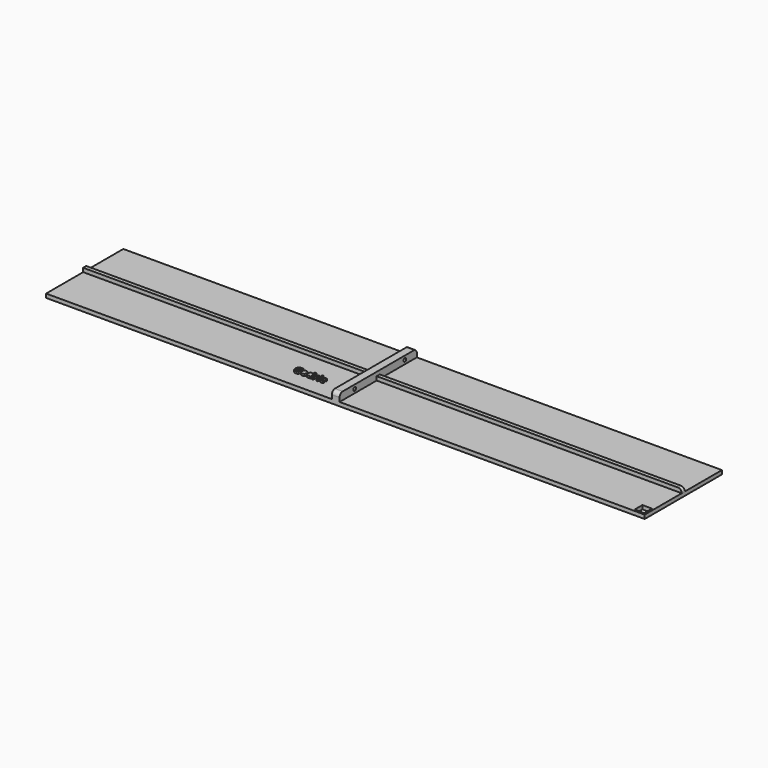
from build123d import *

# Parameters (mm, degrees)
F1_DEPTH     = 2
F0_W         = 0.7426452889
F0_H         = 2.7227729689
F0_W_2       = 5
F0_H_2       = 5
F2_DEPTH     = 4
F3_DEPTH     = 6
F4_R         = 0.885
F5_DEPTH     = 30.275
F6_R         = 2
F0_TEXT_SIZE = 4.9873345738
F7_DEPTH     = 3


# Not quite as in the source:
# - Text() gives the source's letters only with a copy of the font that has no kerning and outlines rounded to 1/6400 em; it was checked with that copy


with BuildPart() as f1:
    # F0 (on Top) → F1 (new body)
    with BuildSketch(Plane.XY):
        Polygon((-87.8959557414, 31.1546225101), (-235.8959557414, 31.1546225101), (-235.8959557414, 7.1546225101), (-234.8959557414, 7.1546225101), (-87.8959557414, 7.1546225101), align=None)
    extrude(amount=F1_DEPTH)



with BuildPart() as f1b:
    # F0 (on Top) → F1, piece 2 (new body)
    with BuildSketch(Plane.XY):
        Polygon((74.1040442586, 31.1546225101), (-83.8959557414, 31.1546225101), (-83.8959557414, 7.1546225101), (64.1040442586, 7.1546225101), (74.1040442586, 7.1546225101), align=None)
    extrude(amount=F1_DEPTH)



with BuildPart() as f1c:
    # F0 (on Top) → F1, piece 3 (new body)
    with BuildSketch(Plane.XY):
        Polygon((-234.8959557414, 5.1546225101), (-235.8959557414, 5.1546225101), (-235.8959557414, -18.8453774899), (-87.8959557414, -18.8453774899), (-87.8959557414, 5.1546225101), align=None)
        with BuildLine():
            add(Edge.make_bspline(
                [(-109.0030381923, -8.150502003), (-108.8425083607, -8.4696134887), (-108.8425083607, -8.8982125536)],
                knots=[0, 0, 0, 1, 1, 1], degree=2))
            add(Edge.make_bspline(
                [(-108.8425083607, -8.8982125536), (-108.8425083607, -9.5629307398), (-109.1931803229, -9.9381497394)],
                knots=[0, 0, 0, 1, 1, 1], degree=2))
            add(Edge.make_bspline(
                [(-109.1931803229, -9.9381497394), (-109.5438522851, -10.3133687389), (-110.16960692, -10.3133687389)],
                knots=[0, 0, 0, 1, 1, 1], degree=2))
            add(Edge.make_bspline(
                [(-110.16960692, -10.3133687389), (-110.5615802466, -10.3133687389), (-110.8612099566, -10.1415394774)],
                knots=[0, 0, 0, 1, 1, 1], degree=2))
            add(Edge.make_bspline(
                [(-110.8612099566, -10.1415394774), (-111.1608396665, -9.969710216), (-111.3213694981, -9.6482609173)],
                knots=[0, 0, 0, 1, 1, 1], degree=2))
            add(Edge.make_bspline(
                [(-111.3213694981, -9.6482609173), (-111.4818993297, -9.3268116185), (-111.4818993297, -8.8982125536)],
                knots=[0, 0, 0, 1, 1, 1], degree=2))
            add(Edge.make_bspline(
                [(-111.4818993297, -8.8982125536), (-111.4818993297, -8.2311565544), (-111.1339548161, -7.8610028165)],
                knots=[0, 0, 0, 1, 1, 1], degree=2))
            add(Edge.make_bspline(
                [(-111.1339548161, -7.8610028165), (-110.7860103024, -7.4908490785), (-110.1548007704, -7.4908490785)],
                knots=[0, 0, 0, 1, 1, 1], degree=2))
            add(Edge.make_bspline(
                [(-110.1548007704, -7.4908490785), (-109.7628274438, -7.4908490785), (-109.4631977338, -7.661119798)],
                knots=[0, 0, 0, 1, 1, 1], degree=2))
            add(Edge.make_bspline(
                [(-109.4631977338, -7.661119798), (-109.1635680239, -7.8313905174), (-109.0030381923, -8.150502003)],
                knots=[0, 0, 0, 1, 1, 1], degree=2))
        make_face(mode=Mode.SUBTRACT)
        with BuildLine():
            Line((-113.5181345237, -8.8935369274), (-113.5181345237, -8.2646652085))
            Line((-113.5181345237, -8.2646652085), (-112.1053161514, -8.2646652085))
            Line((-112.1053161514, -8.2646652085), (-112.1053161514, -10.1107582719))
            add(Edge.make_bspline(
                [(-112.1053161514, -10.1107582719), (-112.4489746744, -10.2229732998), (-112.752111104, -10.2681710194)],
                knots=[0, 0, 0, 1, 1, 1], degree=2))
            add(Edge.make_bspline(
                [(-112.752111104, -10.2681710194), (-113.0552475335, -10.3133687389), (-113.3716315706, -10.3133687389)],
                knots=[0, 0, 0, 1, 1, 1], degree=2))
            add(Edge.make_bspline(
                [(-113.3716315706, -10.3133687389), (-114.1773978127, -10.3133687389), (-114.602490158, -9.8395719544)],
                knots=[0, 0, 0, 1, 1, 1], degree=2))
            add(Edge.make_bspline(
                [(-114.602490158, -9.8395719544), (-115.0275825033, -9.3657751699), (-115.0275825033, -8.478964741)],
                knots=[0, 0, 0, 1, 1, 1], degree=2))
            add(Edge.make_bspline(
                [(-115.0275825033, -8.478964741), (-115.0275825033, -7.6170909849), (-114.5343039431, -7.1351118546)],
                knots=[0, 0, 0, 1, 1, 1], degree=2))
            add(Edge.make_bspline(
                [(-114.5343039431, -7.1351118546), (-114.0410253829, -6.6531327243), (-113.1674625615, -6.6531327243)],
                knots=[0, 0, 0, 1, 1, 1], degree=2))
            add(Edge.make_bspline(
                [(-113.1674625615, -6.6531327243), (-112.6188557583, -6.6531327243), (-112.1099917776, -6.872107883)],
                knots=[0, 0, 0, 1, 1, 1], degree=2))
            Line((-112.1099917776, -6.872107883), (-112.3609170483, -7.476042929))
            add(Edge.make_bspline(
                [(-112.3609170483, -7.476042929), (-112.7505525619, -7.2812251722), (-113.1721381876, -7.2812251722)],
                knots=[0, 0, 0, 1, 1, 1], degree=2))
            add(Edge.make_bspline(
                [(-113.1721381876, -7.2812251722), (-113.6615203927, -7.2812251722), (-113.9560848409, -7.6100775457)],
                knots=[0, 0, 0, 1, 1, 1], degree=2))
            add(Edge.make_bspline(
                [(-113.9560848409, -7.6100775457), (-114.2506492892, -7.9389299192), (-114.2506492892, -8.4937708905)],
                knots=[0, 0, 0, 1, 1, 1], degree=2))
            add(Edge.make_bspline(
                [(-114.2506492892, -8.4937708905), (-114.2506492892, -9.0735485347), (-114.0133612614, -9.3790227774)],
                knots=[0, 0, 0, 1, 1, 1], degree=2))
            add(Edge.make_bspline(
                [(-114.0133612614, -9.3790227774), (-113.7760732337, -9.68449702), (-113.3233167669, -9.68449702)],
                knots=[0, 0, 0, 1, 1, 1], degree=2))
            add(Edge.make_bspline(
                [(-113.3233167669, -9.68449702), (-113.0864183746, -9.68449702), (-112.8432858142, -9.6361822163)],
                knots=[0, 0, 0, 1, 1, 1], degree=2))
            Line((-112.8432858142, -9.6361822163), (-112.8432858142, -8.8935369274))
            Line((-112.8432858142, -8.8935369274), (-113.5181345237, -8.8935369274))
        make_face(mode=Mode.SUBTRACT)
        with BuildLine():
            add(Edge.make_bspline(
                [(-104.0215481511, -7.6307282279), (-103.8060797121, -7.4908490785), (-103.5528166283, -7.4908490785)],
                knots=[0, 0, 0, 1, 1, 1], degree=2))
            add(Edge.make_bspline(
                [(-103.5528166283, -7.4908490785), (-103.401638049, -7.4908490785), (-103.3018913576, -7.5126686673)],
                knots=[0, 0, 0, 1, 1, 1], degree=2))
            Line((-103.3018913576, -7.5126686673), (-103.3579988715, -8.2085576946))
            add(Edge.make_bspline(
                [(-103.3579988715, -8.2085576946), (-103.4483943107, -8.1844002927), (-103.5769740301, -8.1844002927)],
                knots=[0, 0, 0, 1, 1, 1], degree=2))
            add(Edge.make_bspline(
                [(-103.5769740301, -8.1844002927), (-103.9323216185, -8.1844002927), (-104.1310357305, -8.3671393486)],
                knots=[0, 0, 0, 1, 1, 1], degree=2))
            add(Edge.make_bspline(
                [(-104.1310357305, -8.3671393486), (-104.3297498424, -8.5498784045), (-104.3297498424, -8.8787307779)],
                knots=[0, 0, 0, 1, 1, 1], degree=2))
            Line((-104.3297498424, -8.8787307779), (-104.3297498424, -10.2642746642))
            Line((-104.3297498424, -10.2642746642), (-105.0723951313, -10.2642746642))
            Line((-105.0723951313, -10.2642746642), (-105.0723951313, -7.5415016953))
            Line((-105.0723951313, -7.5415016953), (-104.5097614497, -7.5415016953))
            Line((-104.5097614497, -7.5415016953), (-104.3998842348, -7.9997130593))
            Line((-104.3998842348, -7.9997130593), (-104.3640377676, -7.9997130593))
            add(Edge.make_bspline(
                [(-104.3640377676, -7.9997130593), (-104.2370165902, -7.7706073773), (-104.0215481511, -7.6307282279)],
                knots=[0, 0, 0, 1, 1, 1], degree=2))
        make_face(mode=Mode.SUBTRACT)
        with Locations((-102.4365108819, -8.9028881798)):
            Rectangle(F0_W, F0_H, mode=Mode.SUBTRACT)
        with BuildLine():
            add(Edge.make_bspline(
                [(-99.7164653616, -10.2693399259), (-99.900373324, -10.3133687389), (-100.1801316227, -10.3133687389)],
                knots=[0, 0, 0, 1, 1, 1], degree=2))
            add(Edge.make_bspline(
                [(-100.1801316227, -10.3133687389), (-101.451122668, -10.3133687389), (-101.451122668, -8.9176943293)],
                knots=[0, 0, 0, 1, 1, 1], degree=2))
            add(Edge.make_bspline(
                [(-101.451122668, -8.9176943293), (-101.451122668, -8.2233638441), (-101.1055159675, -7.8571064613)],
                knots=[0, 0, 0, 1, 1, 1], degree=2))
            add(Edge.make_bspline(
                [(-101.1055159675, -7.8571064613), (-100.759909267, -7.4908490785), (-100.1146728565, -7.4908490785)],
                knots=[0, 0, 0, 1, 1, 1], degree=2))
            add(Edge.make_bspline(
                [(-100.1146728565, -7.4908490785), (-99.642434614, -7.4908490785), (-99.2668259789, -7.675536312)],
                knots=[0, 0, 0, 1, 1, 1], degree=2))
            Line((-99.2668259789, -7.675536312), (-99.4865804086, -8.25063833))
            add(Edge.make_bspline(
                [(-99.4865804086, -8.25063833), (-99.6619163897, -8.1797246666), (-99.8127053334, -8.134526947)],
                knots=[0, 0, 0, 1, 1, 1], degree=2))
            add(Edge.make_bspline(
                [(-99.8127053334, -8.134526947), (-99.9634942772, -8.0893292274), (-100.1146728565, -8.0893292274)],
                knots=[0, 0, 0, 1, 1, 1], degree=2))
            add(Edge.make_bspline(
                [(-100.1146728565, -8.0893292274), (-100.6944505007, -8.0893292274), (-100.6944505007, -8.9130187031)],
                knots=[0, 0, 0, 1, 1, 1], degree=2))
            add(Edge.make_bspline(
                [(-100.6944505007, -8.9130187031), (-100.6944505007, -9.711771506), (-100.1146728565, -9.711771506)],
                knots=[0, 0, 0, 1, 1, 1], degree=2))
            add(Edge.make_bspline(
                [(-100.1146728565, -9.711771506), (-99.900373324, -9.711771506), (-99.7176342681, -9.6544950855)],
                knots=[0, 0, 0, 1, 1, 1], degree=2))
            add(Edge.make_bspline(
                [(-99.7176342681, -9.6544950855), (-99.5348952122, -9.597218665), (-99.3525457919, -9.4748731137)],
                knots=[0, 0, 0, 1, 1, 1], degree=2))
            Line((-99.3525457919, -9.4748731137), (-99.3525457919, -10.1107582719))
            add(Edge.make_bspline(
                [(-99.3525457919, -10.1107582719), (-99.5325573992, -10.2253111129), (-99.7164653616, -10.2693399259)],
                knots=[0, 0, 0, 1, 1, 1], degree=2))
        make_face(mode=Mode.SUBTRACT)
        with BuildLine():
            add(Edge.make_bspline(
                [(-106.5943114473, -9.9112648889), (-106.8475745312, -10.3133687389), (-107.3665690352, -10.3133687389)],
                knots=[0, 0, 0, 1, 1, 1], degree=2))
            add(Edge.make_bspline(
                [(-107.3665690352, -10.3133687389), (-107.845820717, -10.3133687389), (-108.119734483, -9.9404875524)],
                knots=[0, 0, 0, 1, 1, 1], degree=2))
            add(Edge.make_bspline(
                [(-108.119734483, -9.9404875524), (-108.393648249, -9.5676063659), (-108.393648249, -8.9075638059)],
                knots=[0, 0, 0, 1, 1, 1], degree=2))
            add(Edge.make_bspline(
                [(-108.393648249, -8.9075638059), (-108.393648249, -8.2381699936), (-108.1150588568, -7.8645095361)],
                knots=[0, 0, 0, 1, 1, 1], degree=2))
            add(Edge.make_bspline(
                [(-108.1150588568, -7.8645095361), (-107.8364694646, -7.4908490785), (-107.3470872596, -7.4908490785)],
                knots=[0, 0, 0, 1, 1, 1], degree=2))
            add(Edge.make_bspline(
                [(-107.3470872596, -7.4908490785), (-106.8327683816, -7.4908490785), (-106.5623613352, -7.8898358445)],
                knots=[0, 0, 0, 1, 1, 1], degree=2))
            Line((-106.5623613352, -7.8898358445), (-106.5382039334, -7.8898358445))
            add(Edge.make_bspline(
                [(-106.5382039334, -7.8898358445), (-106.5943114473, -7.5851408728), (-106.5943114473, -7.3466839385)],
                knots=[0, 0, 0, 1, 1, 1], degree=2))
            Line((-106.5943114473, -7.3466839385), (-106.5943114473, -6.4746796591))
            Line((-106.5943114473, -6.4746796591), (-105.8493283454, -6.4746796591))
            Line((-105.8493283454, -6.4746796591), (-105.8493283454, -10.2642746642))
            Line((-105.8493283454, -10.2642746642), (-106.4189754662, -10.2642746642))
            Line((-106.4189754662, -10.2642746642), (-106.5623613352, -9.9112648889))
            Line((-106.5623613352, -9.9112648889), (-106.5943114473, -9.9112648889))
        make_face(mode=Mode.SUBTRACT)
        with BuildLine():
            add(Edge.make_bspline(
                [(-102.4353419754, -7.2032980695), (-102.8397836385, -7.2032980695), (-102.8397836385, -6.8378199578)],
                knots=[0, 0, 0, 1, 1, 1], degree=2))
            add(Edge.make_bspline(
                [(-102.8397836385, -6.8378199578), (-102.8397836385, -6.4746796591), (-102.4353419754, -6.4746796591)],
                knots=[0, 0, 0, 1, 1, 1], degree=2))
            add(Edge.make_bspline(
                [(-102.4353419754, -6.4746796591), (-102.0309003123, -6.4746796591), (-102.0309003123, -6.8378199578)],
                knots=[0, 0, 0, 1, 1, 1], degree=2))
            add(Edge.make_bspline(
                [(-102.0309003123, -6.8378199578), (-102.0309003123, -7.0108181258), (-102.1318159103, -7.1070580977)],
                knots=[0, 0, 0, 1, 1, 1], degree=2))
            add(Edge.make_bspline(
                [(-102.1318159103, -7.1070580977), (-102.2327315083, -7.2032980695), (-102.4353419754, -7.2032980695)],
                knots=[0, 0, 0, 1, 1, 1], degree=2))
        make_face(mode=Mode.SUBTRACT)
    extrude(amount=F1_DEPTH)


with BuildPart() as f1d:
    # F0 (on Top) → F1, piece 4 (new body)
    with BuildSketch(Plane.XY):
        Polygon((64.1040442586, 5.1546225101), (-83.8959557414, 5.1546225101), (-83.8959557414, -18.8453774899), (74.1040442586, -18.8453774899), (74.1040442586, 5.1546225101), align=None)
        with Locations((70.6040442586, -15.3453774899)):
            Rectangle(F0_W_2, F0_H_2, mode=Mode.SUBTRACT)
    extrude(amount=F1_DEPTH)


with BuildPart() as f1_1:
    add(f1.part)

    add(f1c.part)  # F2 merges F1c
    # F0 (on Top) → F2 (join)
    with BuildSketch(Plane.XY):
        Polygon((-234.8959557414, 7.1546225101), (-235.8959557414, 7.1546225101), (-235.8959557414, 5.1546225101), (-234.8959557414, 5.1546225101), (-87.8959557414, 5.1546225101), (-87.8959557414, 7.1546225101), align=None)
    extrude(amount=F2_DEPTH)



with BuildPart() as f1b_1:
    add(f1b.part)

    add(f1d.part)  # F2#2 merges F1d
    # F0 (on Top) → F2, piece 2 (join)
    with BuildSketch(Plane.XY):
        Polygon((64.1040442586, 7.1546225101), (-83.8959557414, 7.1546225101), (-83.8959557414, 5.1546225101), (64.1040442586, 5.1546225101), (74.1040442586, 5.1546225101), (74.1040442586, 7.1546225101), align=None)
    extrude(amount=F2_DEPTH)


with BuildPart() as f1_2:
    add(f1_1.part)

    add(f1b_1.part)  # F3 merges F1b
    # F0 (on Top) → F3 (join)
    with BuildSketch(Plane.XY):
        Polygon((-83.8959557414, 31.1546225101), (-87.8959557414, 31.1546225101), (-87.8959557414, 7.1546225101), (-87.8959557414, 5.1546225101), (-87.8959557414, -18.8453774899), (-83.8959557414, -18.8453774899), (-83.8959557414, 5.1546225101), (-83.8959557414, 7.1546225101), align=None)
    extrude(amount=F3_DEPTH)

    # F4 (on face) → F5 (cut)
    with BuildSketch(Plane(origin=(-87.8959557414, 0, 0), x_dir=(0, -1, 0), z_dir=(-1, 0, 0))):
        with Locations((-23.3864132315, 4.00000019)):
            Circle(F4_R)
        with Locations((9.0922731906, 4.00000019)):
            Circle(F4_R)
    extrude(amount=-F5_DEPTH, mode=Mode.SUBTRACT)

    # F6
    f6_edges = [f1_2.edges().sort_by_distance(p)[0] for p in [
        (-85.895956, 31.154623, 6),
        (-85.895956, -18.845377, 6),
        (74.104044, 6.154623, 4),
    ]]
    fillet(f6_edges, radius=F6_R)

    # F0 (on Top) → F7 (join)
    with BuildSketch(Plane.XY):
        with BuildLine():
            add(Edge.make_bspline(
                [(-110.5935303587, -8.2903811524), (-110.7252271623, -8.4914330774), (-110.7252271623, -8.8982125536)],
                knots=[0, 0, 0, 1, 1, 1], degree=2))
            add(Edge.make_bspline(
                [(-110.7252271623, -8.8982125536), (-110.7252271623, -9.3026542167), (-110.5923614522, -9.5095506744)],
                knots=[0, 0, 0, 1, 1, 1], degree=2))
            add(Edge.make_bspline(
                [(-110.5923614522, -9.5095506744), (-110.4594957421, -9.7164471321), (-110.1602556676, -9.7164471321)],
                knots=[0, 0, 0, 1, 1, 1], degree=2))
            add(Edge.make_bspline(
                [(-110.1602556676, -9.7164471321), (-109.8625741353, -9.7164471321), (-109.7324358737, -9.510719581)],
                knots=[0, 0, 0, 1, 1, 1], degree=2))
            add(Edge.make_bspline(
                [(-109.7324358737, -9.510719581), (-109.6022976122, -9.3049920298), (-109.6022976122, -8.8982125536)],
                knots=[0, 0, 0, 1, 1, 1], degree=2))
            add(Edge.make_bspline(
                [(-109.6022976122, -8.8982125536), (-109.6022976122, -8.4937708905), (-109.7336047803, -8.291550059)],
                knots=[0, 0, 0, 1, 1, 1], degree=2))
            add(Edge.make_bspline(
                [(-109.7336047803, -8.291550059), (-109.8649119483, -8.0893292274), (-110.1649312938, -8.0893292274)],
                knots=[0, 0, 0, 1, 1, 1], degree=2))
            add(Edge.make_bspline(
                [(-110.1649312938, -8.0893292274), (-110.4618335551, -8.0893292274), (-110.5935303587, -8.2903811524)],
                knots=[0, 0, 0, 1, 1, 1], degree=2))
        make_face()
        with BuildLine():
            add(Edge.make_bspline(
                [(-107.502941465, -9.5200708333), (-107.3642312222, -9.7211227583), (-107.1055132411, -9.7211227583)],
                knots=[0, 0, 0, 1, 1, 1], degree=2))
            add(Edge.make_bspline(
                [(-107.1055132411, -9.7211227583), (-106.8210793162, -9.7211227583), (-106.6882136061, -9.555527665)],
                knots=[0, 0, 0, 1, 1, 1], degree=2))
            add(Edge.make_bspline(
                [(-106.6882136061, -9.555527665), (-106.555347896, -9.3899325717), (-106.5428795595, -8.9932836189)],
                knots=[0, 0, 0, 1, 1, 1], degree=2))
            Line((-106.5428795595, -8.9932836189), (-106.5428795595, -8.9130187031))
            add(Edge.make_bspline(
                [(-106.5428795595, -8.9130187031), (-106.5428795595, -8.4742891148), (-106.6780830827, -8.2845366197)],
                knots=[0, 0, 0, 1, 1, 1], degree=2))
            add(Edge.make_bspline(
                [(-106.6780830827, -8.2845366197), (-106.813286606, -8.0947841246), (-107.1179815776, -8.0947841246)],
                knots=[0, 0, 0, 1, 1, 1], degree=2))
            add(Edge.make_bspline(
                [(-107.1179815776, -8.0947841246), (-107.3665690352, -8.0947841246), (-107.5041103715, -8.3051873019)],
                knots=[0, 0, 0, 1, 1, 1], degree=2))
            add(Edge.make_bspline(
                [(-107.5041103715, -8.3051873019), (-107.6416517078, -8.5155904793), (-107.6416517078, -8.9176943293)],
                knots=[0, 0, 0, 1, 1, 1], degree=2))
            add(Edge.make_bspline(
                [(-107.6416517078, -8.9176943293), (-107.6416517078, -9.3190189083), (-107.502941465, -9.5200708333)],
                knots=[0, 0, 0, 1, 1, 1], degree=2))
        make_face()
        with Locations((-115.3174713254, -10.2642746642)):
            Text('Godric', F0_TEXT_SIZE, font='Open Sans', font_style=FontStyle.BOLD, text_align=(TextAlign.LEFT, TextAlign.BOTTOM))
    extrude(amount=F7_DEPTH)


solid = f1_2.part
